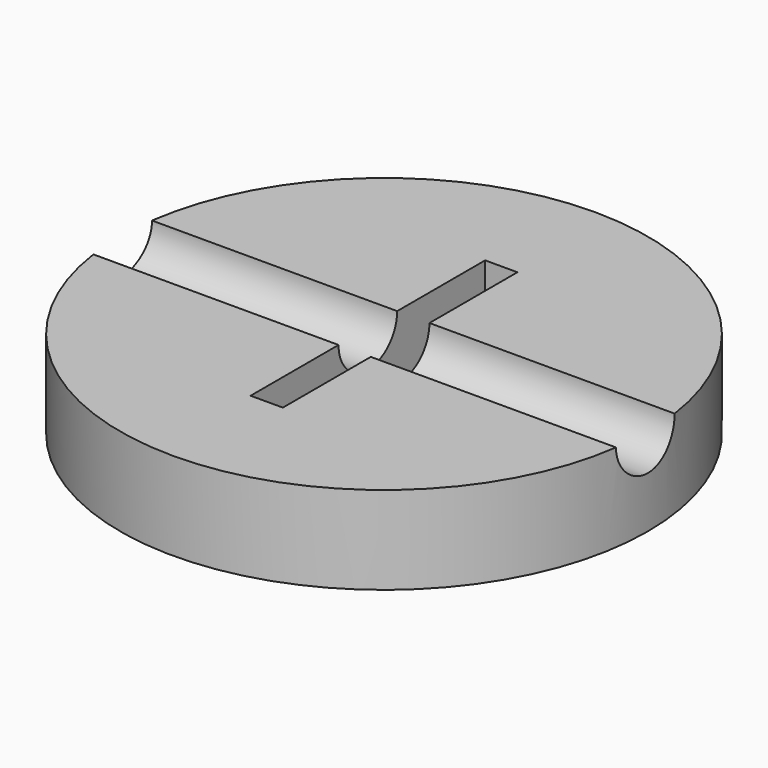
from build123d import *

# Parameters (mm, degrees)
F0_R     = 9
F1_DEPTH = 3
F2_R     = 5.5
F3_DEPTH = 1
F4_R     = 1.25
F5_DEPTH = 9
F6_W     = 1.1
F6_H     = 3.75
F6_H_2   = 2.5
F7_DEPTH = 4.001


# Not quite as in the source:
# - a feature names something its author has since deleted; it is built from what else it names


with BuildPart() as f1:
    # F0 (on Top) → F1 (new body)
    with BuildSketch(Plane.XY):
        Circle(F0_R)
    extrude(amount=-F1_DEPTH)

    # F2 (on face) → F3 (join)
    with BuildSketch(Plane(origin=(0, 0, -3), x_dir=(1, 0, 0), z_dir=(0, 0, -1))):
        Circle(F2_R)
    extrude(amount=F3_DEPTH)

    # F4 (on Right) → F5 (cut, symmetric)
    with BuildSketch(Plane.YZ):
        Circle(F4_R)
    extrude(amount=F5_DEPTH, both=True, mode=Mode.SUBTRACT)

    # F6 (on face) → F7 (cut, through all)
    with BuildSketch(Plane.XY):
        with Locations((0, -3.125)):
            Rectangle(F6_W, F6_H)
        Rectangle(F6_W, F6_H_2)
        with Locations((0, 3.125)):
            Rectangle(F6_W, F6_H)
    extrude(amount=-F7_DEPTH, mode=Mode.SUBTRACT)


solid = f1.part
